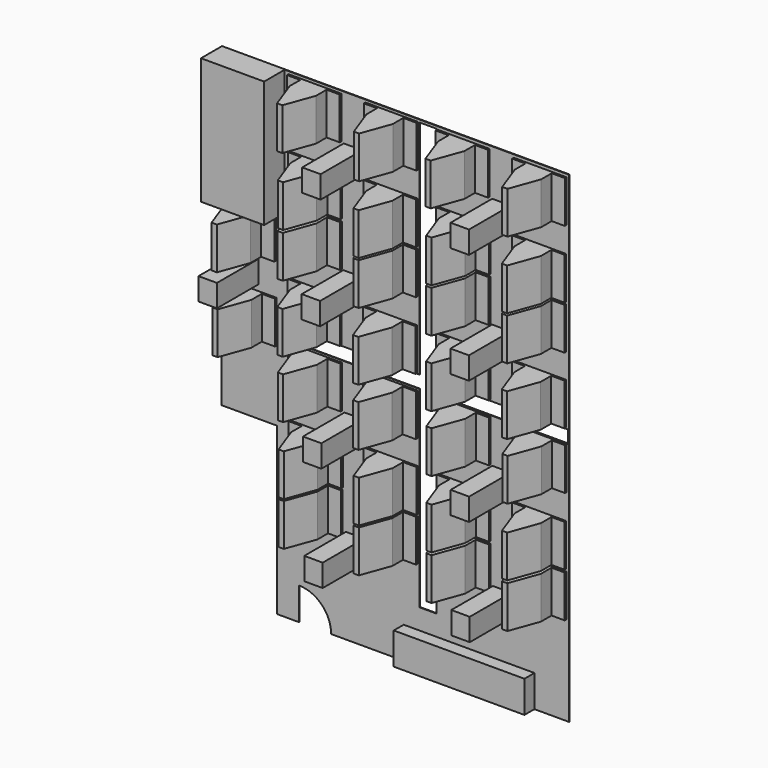
from build123d import *

# Parameters (mm, degrees)
F0_W      = 700
F0_H      = 850
F1_DEPTH  = 25
F0_W_2    = 2400
F0_H_2    = 4800
F2_DEPTH  = 1000
F0_W_3    = 1000
F0_H_3    = 1600
F3_DEPTH  = 1700
F0_W_4    = 500
F4_DEPTH  = 100
F5_DEPTH  = 2000
F6_SIZE2  = 1098.9909677818
F6_SIZE   = 400
F7_SIZE2  = 1098.9909677818
F7_SIZE   = 400
F8_SIZE2  = 1098.9909677818
F8_SIZE   = 400
F9_SIZE2  = 1098.9909677818
F9_SIZE   = 400
F10_SIZE2 = 1098.9909677818
F10_SIZE  = 400
F11_SIZE2 = 1098.9909677818
F11_SIZE  = 400
F12_SIZE2 = 1098.9909677818
F12_SIZE  = 400
F13_SIZE2 = 1098.9909677818
F13_SIZE  = 400
F14_SIZE2 = 1098.9909677818
F14_SIZE  = 400
F15_SIZE2 = 1098.9909677818
F15_SIZE  = 400
F16_SIZE2 = 1098.9909677818
F16_SIZE  = 400
F17_SIZE2 = 1098.9909677818
F17_SIZE  = 400
F18_SIZE2 = 1098.9909677818
F18_SIZE  = 400
F19_SIZE2 = 1098.9909677818
F19_SIZE  = 400
F20_SIZE2 = 1098.9909677818
F20_SIZE  = 400
F21_SIZE2 = 1098.9909677818
F21_SIZE  = 400
F22_SIZE2 = 1098.9909677818
F22_SIZE  = 400
F23_SIZE2 = 1098.9909677818
F23_SIZE  = 400
F24_SIZE2 = 1098.9909677818
F24_SIZE  = 400
F25_SIZE2 = 1098.9909677818
F25_SIZE  = 400
F26_SIZE2 = 1098.9909677818
F26_SIZE  = 400
F27_SIZE2 = 1098.9909677818
F27_SIZE  = 400
F28_SIZE2 = 1098.9909677818
F28_SIZE  = 400
F29_SIZE2 = 1098.9909677818
F29_SIZE  = 400
F30_SIZE2 = 1098.9909677818
F30_SIZE  = 400
F31_SIZE2 = 1098.9909677818
F31_SIZE  = 400
F32_SIZE2 = 1098.9909677818
F32_SIZE  = 400
F33_SIZE2 = 1098.9909677818
F33_SIZE  = 400
F34_SIZE2 = 1098.9909677818
F34_SIZE  = 400
F35_SIZE2 = 1098.9909677818
F35_SIZE  = 400
F36_DEPTH = 500


# Not quite as in the source:
# - ends of sketch curves that miss each other by under 0.0002 mm in the source are joined


with BuildPart() as f1:
    # F0 (on Front) → F1 (new body)
    with BuildSketch(Plane.XZ):
        Polygon((1572.6447105408, -7800), (6600, -7800), (6600, 7800), (-4200, 7800), (-4200, 3000), (-6600, 3000), (-6600, -4200), (-4500, -4200), (-4500, -7800), (912.9041433334, -7800), (912.9041433334, -1212.2844457626), (-4460.7768058777, -1212.2844457626), (-4460.7768058777, -732.8954935074), (912.9041433334, -732.8954935074), (912.9041433334, 7702.3966789246), (1572.6447105408, 7702.3966789246), (1572.6447105408, -732.8954935074), (6553.6727905273, -732.8954935074), (6553.6727905273, -1212.2844457626), (1572.6447105408, -1212.2844457626), align=None)
        Polygon((-3994.2376494408, -7120.8878244673), (-3994.2376494408, -5520.8878244673), (-3494.2376494408, -5520.8878244673), (-2494.2376494408, -5520.8878244673), (-1994.2376494408, -5520.8878244673), (-1994.2376494408, -7120.8878244672), (-2494.2376494408, -7120.8878244673), (-3494.2376494408, -7120.8878244673), align=None, mode=Mode.SUBTRACT)
        with Locations((-1526.1505961418, -7324.3477548872)):
            Rectangle(F0_W, F0_H, mode=Mode.SUBTRACT)
        Polygon((-1145.9731936455, -7079.6481336866), (-1145.9731936455, -5479.6481336866), (-645.9731936455, -5479.6481336866), (354.0268063545, -5479.6481336866), (854.0268063545, -5479.6481336866), (854.0268063545, -7079.6481336866), (354.0268063545, -7079.6481336866), (-645.9731936455, -7079.6481336866), align=None, mode=Mode.SUBTRACT)
        Polygon((-3992.9438710213, -5456.5259184156), (-3992.9438710213, -3856.5259184156), (-3492.9438710213, -3856.5259184156), (-2492.9438710213, -3856.5259184156), (-1992.9438710213, -3856.5259184156), (-1992.9438710213, -5456.5259184156), (-2492.9438710213, -5456.5259184156), (-3492.9438710213, -5456.5259184156), align=None, mode=Mode.SUBTRACT)
        Polygon((-1141.2078619003, -5410.0331033979), (-1141.2078619003, -3810.0331033979), (-641.2078619003, -3810.0331033979), (358.7921380997, -3810.0331033979), (858.7921380997, -3810.0331033979), (858.7921380997, -5410.0331033979), (358.7921380997, -5410.0331033979), (-641.2078619003, -5410.0331033979), align=None, mode=Mode.SUBTRACT)
        Polygon((-4019.9106812477, -2890.570470265), (-4019.9106812477, -1290.570470265), (-3519.9106812477, -1290.570470265), (-2519.9106812477, -1290.570470265), (-2019.9106812477, -1290.570470265), (-2019.9106812477, -2890.570470265), (-2519.9106812477, -2890.570470265), (-3519.9106812477, -2890.570470265), align=None, mode=Mode.SUBTRACT)
        with Locations((-1576.4804005623, -3349.6995176588)):
            Rectangle(F0_W, F0_H, mode=Mode.SUBTRACT)
        Polygon((-1156.9433391094, -2887.6043524061), (-1156.9433391094, -1287.6043524061), (-656.9433391094, -1287.6043524061), (343.0566608906, -1287.6043524061), (843.0566608906, -1287.6043524061), (843.0566608906, -2887.6043524061), (343.0566608906, -2887.6043524061), (-656.9433391094, -2887.6043524061), align=None, mode=Mode.SUBTRACT)
        Polygon((1618.3778047562, -7106.9164276123), (1618.3778047562, -5506.9164276123), (2118.3778047562, -5506.9164276123), (3118.3778047562, -5506.9164276123), (3618.3778047562, -5506.9164276123), (3618.3778047562, -7106.9164276123), (3118.3778047562, -7106.9164276123), (2118.3778047562, -7106.9164276123), align=None, mode=Mode.SUBTRACT)
        with Locations((4060.2538347244, -7318.5946464539)):
            Rectangle(F0_W, F0_H, mode=Mode.SUBTRACT)
        Polygon((4496.6648817062, -7108.0596923828), (4496.6648817062, -5508.0596923828), (4996.6648817062, -5508.0596923828), (5996.6648817062, -5508.0596923828), (6496.6648817062, -5508.0596923828), (6496.6648817062, -7108.0596923828), (5996.6648817062, -7108.0596923828), (4996.6648817062, -7108.0596923828), align=None, mode=Mode.SUBTRACT)
        Polygon((1619.6102023125, -5414.4440855299), (1619.6102023125, -3814.4440855299), (2119.6102023125, -3814.4440855299), (3119.6102023125, -3814.4440855299), (3619.6102023125, -3814.4440855299), (3619.6102023125, -5414.4440855299), (3119.6102023125, -5414.4440855299), (2119.6102023125, -5414.4440855299), align=None, mode=Mode.SUBTRACT)
        Polygon((1618.7955260277, -2860.111781529), (1618.7955260277, -1260.111781529), (2118.7955260277, -1260.111781529), (3118.7955260277, -1260.111781529), (3618.7955260277, -1260.111781529), (3618.7955260277, -2860.111781529), (3118.7955260277, -2860.111781529), (2118.7955260277, -2860.111781529), align=None, mode=Mode.SUBTRACT)
        Polygon((4494.5926785469, -5414.4440855299), (4494.5926785469, -3814.4440855299), (4994.5926785469, -3814.4440855299), (5994.5926785469, -3814.4440855299), (6494.5926785469, -3814.4440855299), (6494.5926785469, -5414.4440855299), (5994.5926785469, -5414.4440855299), (4994.5926785469, -5414.4440855299), align=None, mode=Mode.SUBTRACT)
        with Locations((4036.0736727715, -3307.617684773)):
            Rectangle(F0_W, F0_H, mode=Mode.SUBTRACT)
        Polygon((4507.9151511192, -2845.5225195204), (4507.9151511192, -1245.5225195204), (5007.9151511192, -1245.5225195204), (6007.9151511192, -1245.5225195204), (6507.9151511192, -1245.5225195204), (6507.9151511192, -2845.5225195204), (6007.9151511192, -2845.5225195204), (5007.9151511192, -2845.5225195204), align=None, mode=Mode.SUBTRACT)
        Polygon((-6509.399998188, -1527.4416472231), (-6509.399998188, 72.5583527769), (-6009.399998188, 72.5583527769), (-5009.399998188, 72.5583527769), (-4509.399998188, 72.5583527769), (-4509.399998188, -1527.4416472231), (-5009.399998188, -1527.4416472231), (-6009.399998188, -1527.4416472231), align=None, mode=Mode.SUBTRACT)
        with Locations((-5544.2499041557, 724.5157454695)):
            Rectangle(F0_W, F0_H, mode=Mode.SUBTRACT)
        Polygon((-6536.3668084145, 1301.1328194823), (-6536.3668084145, 2901.1328194823), (-6036.3668084145, 2901.1328194823), (-5036.3668084145, 2901.1328194823), (-4536.3668084145, 2901.1328194823), (-4536.3668084145, 1301.1328194823), (-5036.3668084145, 1301.1328194823), (-6036.3668084145, 1301.1328194823), align=None, mode=Mode.SUBTRACT)
        Polygon((-4039.3263801932, -709.6339430128), (-4039.3263801932, 890.3660569872), (-3539.3263801932, 890.3660569872), (-2539.3263801932, 890.3660569872), (-2039.3263801932, 890.3660569872), (-2039.3263801932, -709.6339430128), (-2539.3263801932, -709.6339430128), (-3539.3263801932, -709.6339430128), align=None, mode=Mode.SUBTRACT)
        Polygon((-1164.3439039588, -709.6339430128), (-1164.3439039588, 890.3660569872), (-664.3439039588, 890.3660569872), (335.6560960412, 890.3660569872), (835.6560960412, 890.3660569872), (835.6560960412, -709.6339430128), (335.6560960412, -709.6339430128), (-664.3439039588, -709.6339430128), align=None, mode=Mode.SUBTRACT)
        Polygon((-4031.7372784019, 1835.5877910342), (-4031.7372784019, 3435.5877910342), (-3531.7372784019, 3435.5877910342), (-2531.7372784019, 3435.5877910342), (-2031.7372784019, 3435.5877910342), (-2031.7372784019, 1835.5877910342), (-2531.7372784019, 1835.5877910342), (-3531.7372784019, 1835.5877910342), align=None, mode=Mode.SUBTRACT)
        with Locations((-1622.8629097342, 1397.1924577441)):
            Rectangle(F0_W, F0_H, mode=Mode.SUBTRACT)
        Polygon((-1151.0214313865, 1859.2876229967), (-1151.0214313865, 3459.2876229967), (-651.0214313865, 3459.2876229967), (348.9785686135, 3459.2876229967), (848.9785686135, 3459.2876229967), (848.9785686135, 1859.2876229967), (348.9785686135, 1859.2876229967), (-651.0214313865, 1859.2876229967), align=None, mode=Mode.SUBTRACT)
        Polygon((-4021.7709541321, 3533.475112915), (-4021.7709541321, 5133.475112915), (-3521.7709541321, 5133.475112915), (-2521.7709541321, 5133.475112915), (-2021.7709541321, 5133.475112915), (-2021.7709541321, 3533.475112915), (-2521.7709541321, 3533.475112915), (-3521.7709541321, 3533.475112915), align=None, mode=Mode.SUBTRACT)
        Polygon((-1146.7884778976, 3533.475112915), (-1146.7884778976, 5133.475112915), (-646.7884778976, 5133.475112915), (353.2115221024, 5133.475112915), (853.2115221024, 5133.475112915), (853.2115221024, 3533.475112915), (353.2115221024, 3533.475112915), (-646.7884778976, 3533.475112915), align=None, mode=Mode.SUBTRACT)
        Polygon((-4048.7377643585, 6099.4305610657), (-4048.7377643585, 7699.4305610657), (-3548.7377643585, 7699.4305610657), (-2548.7377643585, 7699.4305610657), (-2048.7377643585, 7699.4305610657), (-2048.7377643585, 6099.4305610657), (-2548.7377643585, 6099.4305610657), (-3548.7377643585, 6099.4305610657), align=None, mode=Mode.SUBTRACT)
        with Locations((-1605.3074836731, 5640.3015136719)):
            Rectangle(F0_W, F0_H, mode=Mode.SUBTRACT)
        Polygon((-1133.4660053253, 6102.3966789246), (-1133.4660053253, 7702.3966789246), (-633.4660053253, 7702.3966789246), (366.5339946747, 7702.3966789246), (866.5339946747, 7702.3966789246), (866.5339946747, 6102.3966789246), (366.5339946747, 6102.3966789246), (-633.4660053253, 6102.3966789246), align=None, mode=Mode.SUBTRACT)
        Polygon((1611.4034548402, -692.1580995832), (1611.4034548402, 907.8419004168), (2111.4034548402, 907.8419004168), (3111.4034548402, 907.8419004168), (3611.4034548402, 907.8419004168), (3611.4034548402, -692.1580995832), (3111.4034548402, -692.1580995832), (2111.4034548402, -692.1580995832), align=None, mode=Mode.SUBTRACT)
        Polygon((1612.0815172791, 1832.3300395693), (1612.0815172791, 3432.3300395693), (2112.0815172791, 3432.3300395693), (3112.0815172791, 3432.3300395693), (3612.0815172791, 3432.3300395693), (3612.0815172791, 1832.3300395693), (3112.0815172791, 1832.3300395693), (2112.0815172791, 1832.3300395693), align=None, mode=Mode.SUBTRACT)
        Polygon((4486.3859310746, -692.1580995832), (4486.3859310746, 907.8419004168), (4986.3859310746, 907.8419004168), (5986.3859310746, 907.8419004168), (6486.3859310746, 907.8419004168), (6486.3859310746, -692.1580995832), (5986.3859310746, -692.1580995832), (4986.3859310746, -692.1580995832), align=None, mode=Mode.SUBTRACT)
        with Locations((4027.8669252992, 1414.6683011736)):
            Rectangle(F0_W, F0_H, mode=Mode.SUBTRACT)
        Polygon((4492.7971258759, 1842.2074351992), (4492.7971258759, 3442.2074351992), (4992.7971258759, 3442.2074351992), (5992.7971258759, 3442.2074351992), (6492.7971258759, 3442.2074351992), (6492.7971258759, 1842.2074351992), (5992.7971258759, 1842.2074351992), (4992.7971258759, 1842.2074351992), align=None, mode=Mode.SUBTRACT)
        Polygon((1615.7647490501, 3517.2454152788), (1615.7647490501, 5117.2454152788), (2115.7647490501, 5117.2454152788), (3115.7647490501, 5117.2454152788), (3615.7647490501, 5117.2454152788), (3615.7647490501, 3517.2454152788), (3115.7647490501, 3517.2454152788), (2115.7647490501, 3517.2454152788), align=None, mode=Mode.SUBTRACT)
        Polygon((1588.7979388237, 6083.2008634295), (1588.7979388237, 7683.2008634295), (2088.7979388237, 7683.2008634295), (3088.7979388237, 7683.2008634295), (3588.7979388237, 7683.2008634295), (3588.7979388237, 6083.2008634295), (3088.7979388237, 6083.2008634295), (2088.7979388237, 6083.2008634295), align=None, mode=Mode.SUBTRACT)
        Polygon((4490.7472252846, 3517.2454152788), (4490.7472252846, 5117.2454152788), (4990.7472252846, 5117.2454152788), (5990.7472252846, 5117.2454152788), (6490.7472252846, 5117.2454152788), (6490.7472252846, 3517.2454152788), (5990.7472252846, 3517.2454152788), (4990.7472252846, 3517.2454152788), align=None, mode=Mode.SUBTRACT)
        with Locations((4032.2282195091, 5624.0718160357)):
            Rectangle(F0_W, F0_H, mode=Mode.SUBTRACT)
        Polygon((4504.0696978569, 6086.1669812884), (4504.0696978569, 7686.1669812884), (5004.0696978569, 7686.1669812884), (6004.0696978569, 7686.1669812884), (6504.0696978569, 7686.1669812884), (6504.0696978569, 6086.1669812884), (6004.0696978569, 6086.1669812884), (5004.0696978569, 6086.1669812884), align=None, mode=Mode.SUBTRACT)
        with BuildLine():
            Line((6599.5193834681, -10499.9999999981), (6600, -7800))
            Line((6600, -7800), (1572.6447105408, -7800))
            Line((1572.6447105408, -7800), (1572.6447105408, -8513.6566162109))
            Line((1572.6447105408, -8513.6566162109), (912.9041433334, -8513.6566162109))
            Line((912.9041433334, -8513.6566162109), (912.9041433334, -7800))
            Line((912.9041433334, -7800), (-4500, -7800))
            Line((-4500, -7800), (-4500, -10499.9999572215))
            Line((-4500, -10499.9999572215), (-3665.2235984802, -10499.9999604386))
            Line((-3665.2235984802, -10499.9999604386), (-3665.2235984802, -9270.2560424805))
            ThreePointArc((-3665.2235984802, -9270.2560424805), (-2795.6633332935, -9630.4396986031), (-2435.4796805221, -10499.999965178))
            Line((-2435.4796805221, -10499.999965178), (322.5403726101, -10499.9999758072))
            Line((322.5403726101, -10499.9999758072), (322.5403726101, -9289.8035049438))
            Line((322.5403726101, -9289.8035049438), (5287.6973150722, -9289.8035049438))
            Line((5287.6973150722, -9289.8035049438), (5287.6973150722, -10499.9999949425))
            Line((5287.6973150722, -10499.9999949425), (6599.5193834681, -10499.9999999981))
        make_face()
    extrude(amount=F1_DEPTH)

    # F0 (on Front) → F2 (join)
    with BuildSketch(Plane.XZ):
        with Locations((-5400, 5400)):
            Rectangle(F0_W_2, F0_H_2)
    extrude(amount=F2_DEPTH)

    # F0 (on Front) → F3 (join)
    with BuildSketch(Plane.XZ):
        with Locations((-3048.7377643585, 6899.4305610657)):
            Rectangle(F0_W_3, F0_H_3)
        with Locations((-133.4660053253, 6902.3966789246)):
            Rectangle(F0_W_3, F0_H_3)
        with Locations((2588.7979388237, 6883.2008634295)):
            Rectangle(F0_W_3, F0_H_3)
        with Locations((5504.0696978569, 6886.1669812884)):
            Rectangle(F0_W_3, F0_H_3)
        with Locations((5490.7472252846, 4317.2454152788)):
            Rectangle(F0_W_3, F0_H_3)
        with Locations((2615.7647490501, 4317.2454152788)):
            Rectangle(F0_W_3, F0_H_3)
        with Locations((2612.0815172791, 2632.3300395693)):
            Rectangle(F0_W_3, F0_H_3)
        with Locations((5492.7971258759, 2642.2074351992)):
            Rectangle(F0_W_3, F0_H_3)
        with Locations((-151.0214313865, 2659.2876229967)):
            Rectangle(F0_W_3, F0_H_3)
        with Locations((-146.7884778976, 4333.475112915)):
            Rectangle(F0_W_3, F0_H_3)
        with Locations((-3021.7709541321, 4333.475112915)):
            Rectangle(F0_W_3, F0_H_3)
        with Locations((-3031.7372784019, 2635.5877910342)):
            Rectangle(F0_W_3, F0_H_3)
        with Locations((-5536.3668084145, 2101.1328194823)):
            Rectangle(F0_W_3, F0_H_3)
        with Locations((-5509.399998188, -727.4416472231)):
            Rectangle(F0_W_3, F0_H_3)
        with Locations((-3039.3263801932, 90.3660569872)):
            Rectangle(F0_W_3, F0_H_3)
        with Locations((-3019.9106812477, -2090.570470265)):
            Rectangle(F0_W_3, F0_H_3)
        with Locations((-156.9433391094, -2087.6043524061)):
            Rectangle(F0_W_3, F0_H_3)
        with Locations((-164.3439039588, 90.3660569872)):
            Rectangle(F0_W_3, F0_H_3)
        with Locations((2611.4034548402, 107.8419004168)):
            Rectangle(F0_W_3, F0_H_3)
        with Locations((2618.7955260277, -2060.111781529)):
            Rectangle(F0_W_3, F0_H_3)
        with Locations((5507.9151511192, -2045.5225195204)):
            Rectangle(F0_W_3, F0_H_3)
        with Locations((5486.3859310746, 107.8419004168)):
            Rectangle(F0_W_3, F0_H_3)
        with Locations((5494.5926785469, -4614.4440855299)):
            Rectangle(F0_W_3, F0_H_3)
        with Locations((5496.6648817062, -6308.0596923828)):
            Rectangle(F0_W_3, F0_H_3)
        with Locations((2618.3778047562, -6306.9164276123)):
            Rectangle(F0_W_3, F0_H_3)
        with Locations((2619.6102023125, -4614.4440855299)):
            Rectangle(F0_W_3, F0_H_3)
        with Locations((-141.2078619003, -4610.0331033979)):
            Rectangle(F0_W_3, F0_H_3)
        with Locations((-145.9731936455, -6279.6481336866)):
            Rectangle(F0_W_3, F0_H_3)
        with Locations((-2994.2376494408, -6320.8878244673)):
            Rectangle(F0_W_3, F0_H_3)
        with Locations((-2992.9438710213, -4656.5259184156)):
            Rectangle(F0_W_3, F0_H_3)
    extrude(amount=F3_DEPTH)

    # F0 (on Front) → F4 (join)
    with BuildSketch(Plane.XZ):
        with Locations((-3798.7377643585, 6899.4305610657)):
            Rectangle(F0_W_4, F0_H_3)
        with Locations((-2298.7377643585, 6899.4305610657)):
            Rectangle(F0_W_4, F0_H_3)
        with Locations((-883.4660053253, 6902.3966789246)):
            Rectangle(F0_W_4, F0_H_3)
        with Locations((616.5339946747, 6902.3966789246)):
            Rectangle(F0_W_4, F0_H_3)
        with Locations((1838.7979388237, 6883.2008634295)):
            Rectangle(F0_W_4, F0_H_3)
        with Locations((3338.7979388237, 6883.2008634295)):
            Rectangle(F0_W_4, F0_H_3)
        with Locations((4754.0696978569, 6886.1669812884)):
            Rectangle(F0_W_4, F0_H_3)
        with Locations((6254.0696978569, 6886.1669812884)):
            Rectangle(F0_W_4, F0_H_3)
        with Locations((4740.7472252846, 4317.2454152788)):
            Rectangle(F0_W_4, F0_H_3)
        with Locations((6240.7472252846, 4317.2454152788)):
            Rectangle(F0_W_4, F0_H_3)
        with Locations((6242.7971258759, 2642.2074351992)):
            Rectangle(F0_W_4, F0_H_3)
        with Locations((4742.7971258759, 2642.2074351992)):
            Rectangle(F0_W_4, F0_H_3)
        with Locations((3365.7647490501, 4317.2454152788)):
            Rectangle(F0_W_4, F0_H_3)
        with Locations((3362.0815172791, 2632.3300395693)):
            Rectangle(F0_W_4, F0_H_3)
        with Locations((1862.0815172791, 2632.3300395693)):
            Rectangle(F0_W_4, F0_H_3)
        with Locations((1865.7647490501, 4317.2454152788)):
            Rectangle(F0_W_4, F0_H_3)
        with Locations((603.2115221024, 4333.475112915)):
            Rectangle(F0_W_4, F0_H_3)
        with Locations((598.9785686135, 2659.2876229967)):
            Rectangle(F0_W_4, F0_H_3)
        with Locations((-901.0214313865, 2659.2876229967)):
            Rectangle(F0_W_4, F0_H_3)
        with Locations((-896.7884778976, 4333.475112915)):
            Rectangle(F0_W_4, F0_H_3)
        with Locations((-2271.7709541321, 4333.475112915)):
            Rectangle(F0_W_4, F0_H_3)
        with Locations((-2281.7372784019, 2635.5877910342)):
            Rectangle(F0_W_4, F0_H_3)
        with Locations((-3781.7372784019, 2635.5877910342)):
            Rectangle(F0_W_4, F0_H_3)
        with Locations((-3771.7709541321, 4333.475112915)):
            Rectangle(F0_W_4, F0_H_3)
        with Locations((-3789.3263801932, 90.3660569872)):
            Rectangle(F0_W_4, F0_H_3)
        with Locations((-2289.3263801932, 90.3660569872)):
            Rectangle(F0_W_4, F0_H_3)
        with Locations((-914.3439039588, 90.3660569872)):
            Rectangle(F0_W_4, F0_H_3)
        with Locations((585.6560960412, 90.3660569872)):
            Rectangle(F0_W_4, F0_H_3)
        with Locations((1861.4034548402, 107.8419004168)):
            Rectangle(F0_W_4, F0_H_3)
        with Locations((3361.4034548402, 107.8419004168)):
            Rectangle(F0_W_4, F0_H_3)
        with Locations((4736.3859310746, 107.8419004168)):
            Rectangle(F0_W_4, F0_H_3)
        with Locations((6236.3859310746, 107.8419004168)):
            Rectangle(F0_W_4, F0_H_3)
        with Locations((6257.9151511192, -2045.5225195204)):
            Rectangle(F0_W_4, F0_H_3)
        with Locations((4757.9151511192, -2045.5225195204)):
            Rectangle(F0_W_4, F0_H_3)
        with Locations((3368.7955260277, -2060.111781529)):
            Rectangle(F0_W_4, F0_H_3)
        with Locations((1868.7955260277, -2060.111781529)):
            Rectangle(F0_W_4, F0_H_3)
        with Locations((593.0566608906, -2087.6043524061)):
            Rectangle(F0_W_4, F0_H_3)
        with Locations((-906.9433391094, -2087.6043524061)):
            Rectangle(F0_W_4, F0_H_3)
        with Locations((-2269.9106812477, -2090.570470265)):
            Rectangle(F0_W_4, F0_H_3)
        with Locations((-3769.9106812477, -2090.570470265)):
            Rectangle(F0_W_4, F0_H_3)
        with Locations((-3742.9438710213, -4656.5259184156)):
            Rectangle(F0_W_4, F0_H_3)
        with Locations((-2242.9438710213, -4656.5259184156)):
            Rectangle(F0_W_4, F0_H_3)
        with Locations((-891.2078619003, -4610.0331033979)):
            Rectangle(F0_W_4, F0_H_3)
        with Locations((608.7921380997, -4610.0331033979)):
            Rectangle(F0_W_4, F0_H_3)
        with Locations((1869.6102023125, -4614.4440855299)):
            Rectangle(F0_W_4, F0_H_3)
        with Locations((3369.6102023125, -4614.4440855299)):
            Rectangle(F0_W_4, F0_H_3)
        with Locations((4744.5926785469, -4614.4440855299)):
            Rectangle(F0_W_4, F0_H_3)
        with Locations((6244.5926785469, -4614.4440855299)):
            Rectangle(F0_W_4, F0_H_3)
        with Locations((6246.6648817062, -6308.0596923828)):
            Rectangle(F0_W_4, F0_H_3)
        with Locations((4746.6648817062, -6308.0596923828)):
            Rectangle(F0_W_4, F0_H_3)
        with Locations((3368.3778047562, -6306.9164276123)):
            Rectangle(F0_W_4, F0_H_3)
        with Locations((1868.3778047562, -6306.9164276123)):
            Rectangle(F0_W_4, F0_H_3)
        with Locations((604.0268063545, -6279.6481336866)):
            Rectangle(F0_W_4, F0_H_3)
        with Locations((-895.9731936455, -6279.6481336866)):
            Rectangle(F0_W_4, F0_H_3)
        with Locations((-2244.2376494408, -6320.8878244673)):
            Rectangle(F0_W_4, F0_H_3)
        with Locations((-3744.2376494408, -6320.8878244673)):
            Rectangle(F0_W_4, F0_H_3)
        with Locations((-4759.399998188, -727.4416472231)):
            Rectangle(F0_W_4, F0_H_3)
        with Locations((-6259.399998188, -727.4416472231)):
            Rectangle(F0_W_4, F0_H_3)
        with Locations((-6286.3668084145, 2101.1328194823)):
            Rectangle(F0_W_4, F0_H_3)
        with Locations((-4786.3668084145, 2101.1328194823)):
            Rectangle(F0_W_4, F0_H_3)
    extrude(amount=F4_DEPTH)

    # F0 (on Front) → F5 (join)
    with BuildSketch(Plane.XZ):
        with Locations((-1605.3074836731, 5640.3015136719)):
            Rectangle(F0_W, F0_H)
        with Locations((4032.2282195091, 5624.0718160357)):
            Rectangle(F0_W, F0_H)
        with Locations((4027.8669252992, 1414.6683011736)):
            Rectangle(F0_W, F0_H)
        with Locations((-1622.8629097342, 1397.1924577441)):
            Rectangle(F0_W, F0_H)
        with Locations((-1576.4804005623, -3349.6995176588)):
            Rectangle(F0_W, F0_H)
        with Locations((4036.0736727715, -3307.617684773)):
            Rectangle(F0_W, F0_H)
        with Locations((4060.2538347244, -7318.5946464539)):
            Rectangle(F0_W, F0_H)
        with Locations((-1526.1505961418, -7324.3477548872)):
            Rectangle(F0_W, F0_H)
        with Locations((-5544.2499041557, 724.5157454695)):
            Rectangle(F0_W, F0_H)
    extrude(amount=F5_DEPTH)

    # F6
    f6_edges = [f1.edges().sort_by_distance(p)[0] for p in [
        (-3548.737764, -1700, 6899.430561),
        (-2548.737764, -1700, 6899.430561),
    ]]
    f6_side = f1.faces().sort_by_distance((-3048.737764, -1700, 6899.430561))[0]
    chamfer(f6_edges, length=F6_SIZE, length2=F6_SIZE2, reference=f6_side)

    # F7
    f7_edges = [f1.edges().sort_by_distance(p)[0] for p in [
        (-633.466005, -1700, 6902.396679),
        (366.533995, -1700, 6902.396679),
    ]]
    f7_side = f1.faces().sort_by_distance((-133.466005, -1700, 6902.396679))[0]
    chamfer(f7_edges, length=F7_SIZE, length2=F7_SIZE2, reference=f7_side)

    # F8
    f8_edges = [f1.edges().sort_by_distance(p)[0] for p in [
        (2088.797939, -1700, 6883.200863),
        (3088.797939, -1700, 6883.200863),
    ]]
    f8_side = f1.faces().sort_by_distance((2588.797939, -1700, 6883.200863))[0]
    chamfer(f8_edges, length=F8_SIZE, length2=F8_SIZE2, reference=f8_side)

    # F9
    f9_edges = [f1.edges().sort_by_distance(p)[0] for p in [
        (5004.069698, -1700, 6886.166981),
        (6004.069698, -1700, 6886.166981),
    ]]
    f9_side = f1.faces().sort_by_distance((5504.069698, -1700, 6886.166981))[0]
    chamfer(f9_edges, length=F9_SIZE, length2=F9_SIZE2, reference=f9_side)

    # F10
    f10_edges = [f1.edges().sort_by_distance(p)[0] for p in [
        (-3521.770954, -1700, 4333.475113),
        (-2521.770954, -1700, 4333.475113),
    ]]
    f10_side = f1.faces().sort_by_distance((-3021.770954, -1700, 4333.475113))[0]
    chamfer(f10_edges, length=F10_SIZE, length2=F10_SIZE2, reference=f10_side)

    # F11
    f11_edges = [f1.edges().sort_by_distance(p)[0] for p in [
        (-646.788478, -1700, 4333.475113),
        (353.211522, -1700, 4333.475113),
    ]]
    f11_side = f1.faces().sort_by_distance((-146.788478, -1700, 4333.475113))[0]
    chamfer(f11_edges, length=F11_SIZE, length2=F11_SIZE2, reference=f11_side)

    # F12
    f12_edges = [f1.edges().sort_by_distance(p)[0] for p in [
        (2115.764749, -1700, 4317.245415),
        (3115.764749, -1700, 4317.245415),
    ]]
    f12_side = f1.faces().sort_by_distance((2615.764749, -1700, 4317.245415))[0]
    chamfer(f12_edges, length=F12_SIZE, length2=F12_SIZE2, reference=f12_side)

    # F13
    f13_edges = [f1.edges().sort_by_distance(p)[0] for p in [
        (4990.747225, -1700, 4317.245415),
        (5990.747225, -1700, 4317.245415),
    ]]
    f13_side = f1.faces().sort_by_distance((5490.747225, -1700, 4317.245415))[0]
    chamfer(f13_edges, length=F13_SIZE, length2=F13_SIZE2, reference=f13_side)

    # F14
    f14_edges = [f1.edges().sort_by_distance(p)[0] for p in [
        (-3531.737278, -1700, 2635.587791),
        (-2531.737278, -1700, 2635.587791),
    ]]
    f14_side = f1.faces().sort_by_distance((-3031.737278, -1700, 2635.587791))[0]
    chamfer(f14_edges, length=F14_SIZE, length2=F14_SIZE2, reference=f14_side)

    # F15
    f15_edges = [f1.edges().sort_by_distance(p)[0] for p in [
        (-651.021431, -1700, 2659.287623),
        (348.978569, -1700, 2659.287623),
    ]]
    f15_side = f1.faces().sort_by_distance((-151.021431, -1700, 2659.287623))[0]
    chamfer(f15_edges, length=F15_SIZE, length2=F15_SIZE2, reference=f15_side)

    # F16
    f16_edges = [f1.edges().sort_by_distance(p)[0] for p in [
        (2112.081517, -1700, 2632.33004),
        (3112.081517, -1700, 2632.33004),
    ]]
    f16_side = f1.faces().sort_by_distance((2612.081517, -1700, 2632.33004))[0]
    chamfer(f16_edges, length=F16_SIZE, length2=F16_SIZE2, reference=f16_side)

    # F17
    f17_edges = [f1.edges().sort_by_distance(p)[0] for p in [
        (4992.797126, -1700, 2642.207435),
        (5992.797126, -1700, 2642.207435),
    ]]
    f17_side = f1.faces().sort_by_distance((5492.797126, -1700, 2642.207435))[0]
    chamfer(f17_edges, length=F17_SIZE, length2=F17_SIZE2, reference=f17_side)

    # F18
    f18_edges = [f1.edges().sort_by_distance(p)[0] for p in [
        (-6036.366808, -1700, 2101.132819),
        (-5036.366808, -1700, 2101.132819),
    ]]
    f18_side = f1.faces().sort_by_distance((-5536.366808, -1700, 2101.132819))[0]
    chamfer(f18_edges, length=F18_SIZE, length2=F18_SIZE2, reference=f18_side)

    # F19
    f19_edges = [f1.edges().sort_by_distance(p)[0] for p in [
        (-6009.399998, -1700, -727.441647),
        (-5009.399998, -1700, -727.441647),
    ]]
    f19_side = f1.faces().sort_by_distance((-5509.399998, -1700, -727.441647))[0]
    chamfer(f19_edges, length=F19_SIZE, length2=F19_SIZE2, reference=f19_side)

    # F20
    f20_edges = [f1.edges().sort_by_distance(p)[0] for p in [
        (-3539.32638, -1700, 90.366057),
        (-2539.32638, -1700, 90.366057),
    ]]
    f20_side = f1.faces().sort_by_distance((-3039.32638, -1700, 90.366057))[0]
    chamfer(f20_edges, length=F20_SIZE, length2=F20_SIZE2, reference=f20_side)

    # F21
    f21_edges = [f1.edges().sort_by_distance(p)[0] for p in [
        (-664.343904, -1700, 90.366057),
        (335.656096, -1700, 90.366057),
    ]]
    f21_side = f1.faces().sort_by_distance((-164.343904, -1700, 90.366057))[0]
    chamfer(f21_edges, length=F21_SIZE, length2=F21_SIZE2, reference=f21_side)

    # F22
    f22_edges = [f1.edges().sort_by_distance(p)[0] for p in [
        (2111.403455, -1700, 107.8419),
        (3111.403455, -1700, 107.8419),
    ]]
    f22_side = f1.faces().sort_by_distance((2611.403455, -1700, 107.8419))[0]
    chamfer(f22_edges, length=F22_SIZE, length2=F22_SIZE2, reference=f22_side)

    # F23
    f23_edges = [f1.edges().sort_by_distance(p)[0] for p in [
        (4986.385931, -1700, 107.8419),
        (5986.385931, -1700, 107.8419),
    ]]
    f23_side = f1.faces().sort_by_distance((5486.385931, -1700, 107.8419))[0]
    chamfer(f23_edges, length=F23_SIZE, length2=F23_SIZE2, reference=f23_side)

    # F24
    f24_edges = [f1.edges().sort_by_distance(p)[0] for p in [
        (-3519.910681, -1700, -2090.57047),
        (-2519.910681, -1700, -2090.57047),
    ]]
    f24_side = f1.faces().sort_by_distance((-3019.910681, -1700, -2090.57047))[0]
    chamfer(f24_edges, length=F24_SIZE, length2=F24_SIZE2, reference=f24_side)

    # F25
    f25_edges = [f1.edges().sort_by_distance(p)[0] for p in [
        (-656.943339, -1700, -2087.604352),
        (343.056661, -1700, -2087.604352),
    ]]
    f25_side = f1.faces().sort_by_distance((-156.943339, -1700, -2087.604352))[0]
    chamfer(f25_edges, length=F25_SIZE, length2=F25_SIZE2, reference=f25_side)

    # F26
    f26_edges = [f1.edges().sort_by_distance(p)[0] for p in [
        (2118.795526, -1700, -2060.111782),
        (3118.795526, -1700, -2060.111782),
    ]]
    f26_side = f1.faces().sort_by_distance((2618.795526, -1700, -2060.111782))[0]
    chamfer(f26_edges, length=F26_SIZE, length2=F26_SIZE2, reference=f26_side)

    # F27
    f27_edges = [f1.edges().sort_by_distance(p)[0] for p in [
        (5007.915151, -1700, -2045.52252),
        (6007.915151, -1700, -2045.52252),
    ]]
    f27_side = f1.faces().sort_by_distance((5507.915151, -1700, -2045.52252))[0]
    chamfer(f27_edges, length=F27_SIZE, length2=F27_SIZE2, reference=f27_side)

    # F28
    f28_edges = [f1.edges().sort_by_distance(p)[0] for p in [
        (-3492.943871, -1700, -4656.525918),
        (-2492.943871, -1700, -4656.525918),
    ]]
    f28_side = f1.faces().sort_by_distance((-2992.943871, -1700, -4656.525918))[0]
    chamfer(f28_edges, length=F28_SIZE, length2=F28_SIZE2, reference=f28_side)

    # F29
    f29_edges = [f1.edges().sort_by_distance(p)[0] for p in [
        (-641.207862, -1700, -4610.033103),
        (358.792138, -1700, -4610.033103),
    ]]
    f29_side = f1.faces().sort_by_distance((-141.207862, -1700, -4610.033103))[0]
    chamfer(f29_edges, length=F29_SIZE, length2=F29_SIZE2, reference=f29_side)

    # F30
    f30_edges = [f1.edges().sort_by_distance(p)[0] for p in [
        (2119.610202, -1700, -4614.444086),
        (3119.610202, -1700, -4614.444086),
    ]]
    f30_side = f1.faces().sort_by_distance((2619.610202, -1700, -4614.444086))[0]
    chamfer(f30_edges, length=F30_SIZE, length2=F30_SIZE2, reference=f30_side)

    # F31
    f31_edges = [f1.edges().sort_by_distance(p)[0] for p in [
        (4994.592679, -1700, -4614.444086),
        (5994.592679, -1700, -4614.444086),
    ]]
    f31_side = f1.faces().sort_by_distance((5494.592679, -1700, -4614.444086))[0]
    chamfer(f31_edges, length=F31_SIZE, length2=F31_SIZE2, reference=f31_side)

    # F32
    f32_edges = [f1.edges().sort_by_distance(p)[0] for p in [
        (-3494.237649, -1700, -6320.887824),
        (-2494.237649, -1700, -6320.887824),
    ]]
    f32_side = f1.faces().sort_by_distance((-2994.237649, -1700, -6320.887824))[0]
    chamfer(f32_edges, length=F32_SIZE, length2=F32_SIZE2, reference=f32_side)

    # F33
    f33_edges = [f1.edges().sort_by_distance(p)[0] for p in [
        (-645.973194, -1700, -6279.648134),
        (354.026806, -1700, -6279.648134),
    ]]
    f33_side = f1.faces().sort_by_distance((-145.973194, -1700, -6279.648134))[0]
    chamfer(f33_edges, length=F33_SIZE, length2=F33_SIZE2, reference=f33_side)

    # F34
    f34_edges = [f1.edges().sort_by_distance(p)[0] for p in [
        (2118.377805, -1700, -6306.916428),
        (3118.377805, -1700, -6306.916428),
    ]]
    f34_side = f1.faces().sort_by_distance((2618.377805, -1700, -6306.916428))[0]
    chamfer(f34_edges, length=F34_SIZE, length2=F34_SIZE2, reference=f34_side)

    # F35
    f35_edges = [f1.edges().sort_by_distance(p)[0] for p in [
        (4996.664882, -1700, -6308.059692),
        (5996.664882, -1700, -6308.059692),
    ]]
    f35_side = f1.faces().sort_by_distance((5496.664882, -1700, -6308.059692))[0]
    chamfer(f35_edges, length=F35_SIZE, length2=F35_SIZE2, reference=f35_side)

    # F0 (on Front) → F36 (join)
    with BuildSketch(Plane.XZ):
        Polygon((322.5403726101, -10499.9999758072), (5287.6973150722, -10499.9999949425), (5287.6973150722, -9289.8035049438), (322.5403726101, -9289.8035049438), align=None)
    extrude(amount=F36_DEPTH)


solid = f1.part
